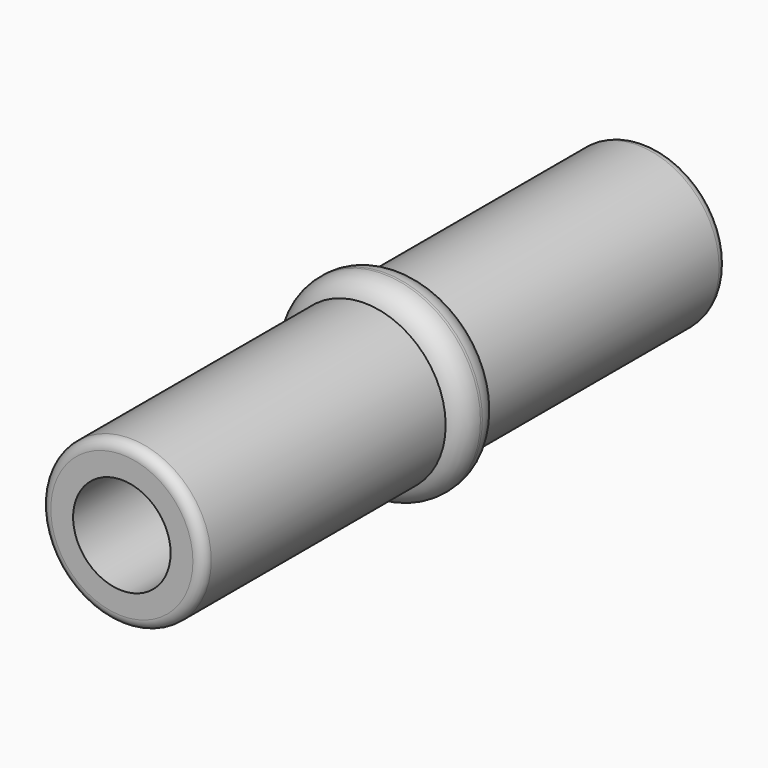
from build123d import *

# Parameters (mm, degrees)
F0_R     = 5
F0_R_2   = 3
F1_DEPTH = 20.162448287
F2_R     = 0.6272281394
F0_R_3   = 6
F3_DEPTH = 1.5


# Not quite as in the source:
# - a fillet or chamfer that OpenCascade refuses, or shapes differently, is made with other operations: its cross-section is extruded or revolved along the edge and cut away or added


with BuildPart() as f1:
    # F0 (on Front) → F1 (new body, symmetric)
    with BuildSketch(Plane.XZ):
        Circle(F0_R)
        Circle(F0_R_2, mode=Mode.SUBTRACT)
    extrude(amount=F1_DEPTH, both=True)

    # F2
    f2_edges = [f1.edges().sort_by_distance(p)[0] for p in [
        (-5, -20.162448, 0),
        (-5, 20.162448, 0),
    ]]
    fillet(f2_edges, radius=F2_R)

    # F0 (on Front) → F3 (join, symmetric)
    with BuildSketch(Plane.XZ):
        Circle(F0_R_3)
        Circle(F0_R, mode=Mode.SUBTRACT)
    extrude(amount=F3_DEPTH, both=True)

    # F4: fillet of radius 1.5182281224 on 2 edges, made by hand

    # F4_s1 → F4_t2 (revolve, cut)
    with BuildSketch(Plane.XY):
        with BuildLine():
            ThreePointArc((5, 1.5), (5.7251151811, 0.9442269358), (6, 0.072955416))
            Line((6, 0.072955416), (6, 1.5))
            Line((6, 1.5), (5, 1.5))
        make_face()
    revolve(axis=Axis((0, 1.5, 0), (0, -1, 0)), mode=Mode.SUBTRACT)

    # F4_s3 → F4_t4 (revolve, cut)
    with BuildSketch(Plane.XY):
        with BuildLine():
            ThreePointArc((6, -0.072955416), (5.7251151811, -0.9442269358), (5, -1.5))
            Line((5, -1.5), (6, -1.5))
            Line((6, -1.5), (6, -0.072955416))
        make_face()
    revolve(axis=Axis((0, -1.5, 0), (0, -1, 0)), mode=Mode.SUBTRACT)


solid = f1.part
